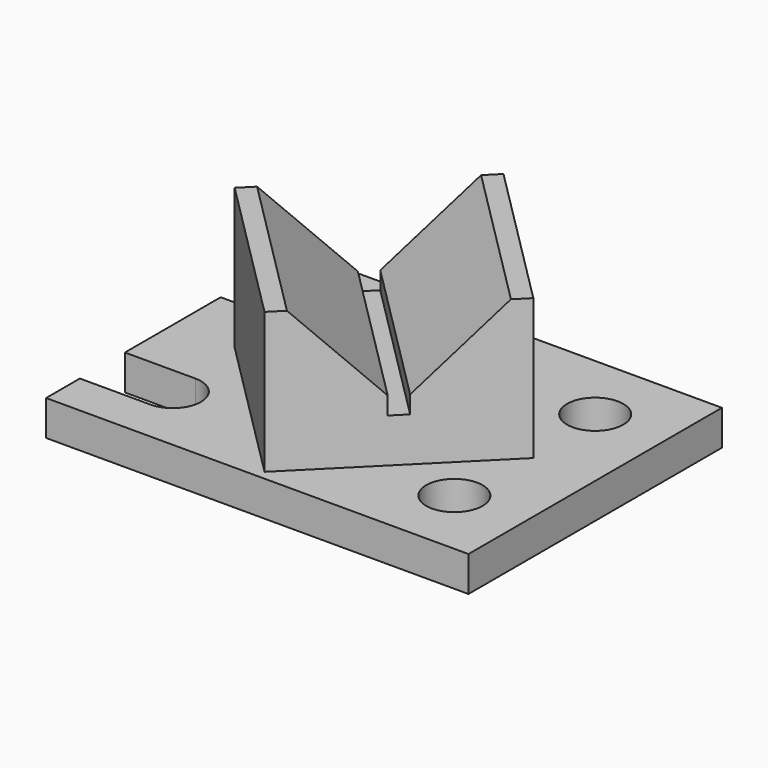
from build123d import *

# Parameters (mm, degrees)
F0_W     = 152.4
F0_H     = 114.3
F1_DEPTH = 12.7
F3_DEPTH = 12.7
F4_R     = 10.16
F5_DEPTH = 12.7
F7_DEPTH = 50.8
F9_DEPTH = 76.2


# Not quite as in the source:
# - a pattern or mirror of a feature is missing from the dataset's text; its kind, count and spacing are read off the source's solid


with BuildPart() as f1:
    # F0 (on Top) → F1 (new body)
    with BuildSketch(Plane.XY):
        Rectangle(F0_W, F0_H)
    extrude(amount=F1_DEPTH)

    # F2 (on face) → F3 (cut, through all)
    with BuildSketch(Plane.XY.offset(12.7)):
        with BuildLine():
            Line((-50.8, -21.59), (-76.2, -21.59))
            Line((-76.2, -21.59), (-76.2, -41.91))
            Line((-76.2, -41.91), (-50.8, -41.91))
            ThreePointArc((-50.8, -41.91), (-40.64, -31.75), (-50.8, -21.59))
        make_face()
    f3 = extrude(amount=-F3_DEPTH, mode=Mode.SUBTRACT)

    # F3_copies: F3 across plane
    add(f3.mirror(Plane.ZX), mode=Mode.SUBTRACT)

    # F4 (on face) → F5 (cut, through all)
    with BuildSketch(Plane.XY.offset(12.7)):
        with Locations((50.8, -31.75)):
            Circle(F4_R)
    f5 = extrude(amount=-F5_DEPTH, mode=Mode.SUBTRACT)

    # F5_copies: F5 across plane
    add(f5.mirror(Plane.ZX), mode=Mode.SUBTRACT)

    # F6 (on face) → F7 (join)
    with BuildSketch(Plane.XY.offset(12.7)):
        Polygon((53.8815367264, 0), (0, 53.8815367264), (-53.8815367264, 0), (0, -53.8815367264), align=None)
    extrude(amount=F7_DEPTH)

    # F8 (on face) → F9 (cut, through all)
    with BuildSketch(Plane(origin=(26.9407683632, -26.9407683632, 0), x_dir=(0.7071067812, 0.7071067812, 0), z_dir=(0.7071067812, -0.7071067812, 0))):
        Polygon((31.75, 63.5), (-31.75, 63.5), (-3.175, 34.925), (-3.175, 28.575), (3.175, 28.575), (3.175, 34.925), align=None)
    extrude(amount=-F9_DEPTH, mode=Mode.SUBTRACT)


solid = f1.part
